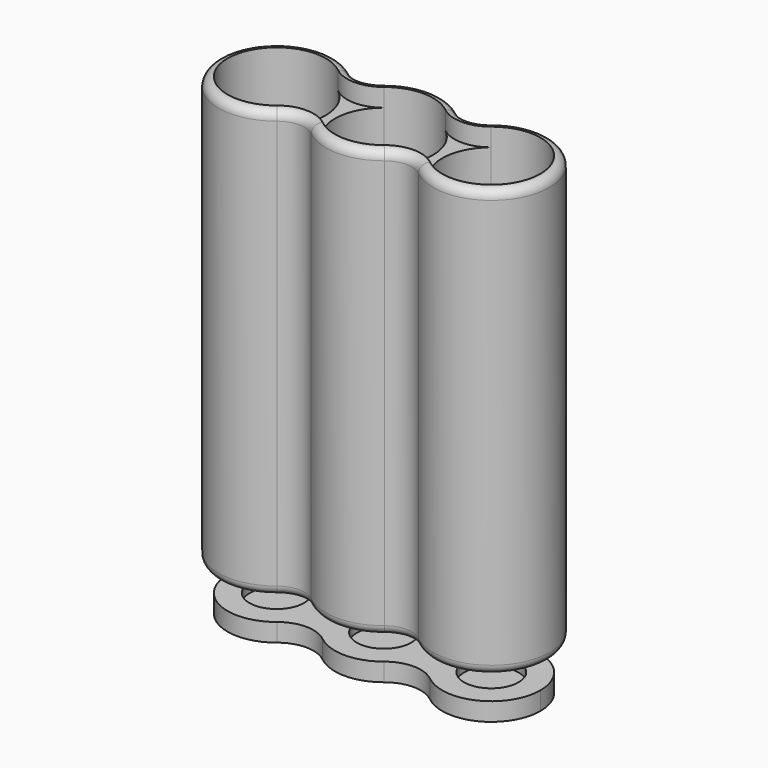
from build123d import *

# Parameters (mm, degrees)
F1_DEPTH = 47
F2_DEPTH = 45
F3_DEPTH = 1
F4_R     = 0.99999
F5_START = -3
F5_DEPTH = 2
F6_R     = 3
F7_DEPTH = 1


# Not quite as in the source:
# - a fillet or chamfer is up to 0.001 mm smaller than in the source, because OpenCascade refuses the exact size


with BuildPart() as f1:
    # F0 (on Top) → F1 (new body)
    with BuildSketch(Plane.XY):
        with BuildLine():
            ThreePointArc((4.0170212766, -4.9823227578), (5.9, -4.3177865506), (7.7829787234, -4.9823227578))
            ThreePointArc((7.7829787234, -4.9823227578), (11.8, -6.4), (15.8170212766, -4.9823227578))
            ThreePointArc((15.8170212766, -4.9823227578), (17.7, -4.3177865506), (19.5829787234, -4.9823227578))
            ThreePointArc((19.5829787234, -4.9823227578), (30, 0), (19.5829787234, 4.9823227578))
            ThreePointArc((19.5829787234, 4.9823227578), (17.7, 4.3177865506), (15.8170212766, 4.9823227578))
            ThreePointArc((15.8170212766, 4.9823227578), (11.8, 6.4), (7.7829787234, 4.9823227578))
            ThreePointArc((7.7829787234, 4.9823227578), (5.9, 4.3177865506), (4.0170212766, 4.9823227578))
            ThreePointArc((4.0170212766, 4.9823227578), (-6.4, 0), (4.0170212766, -4.9823227578))
        make_face()
        with BuildLine():
            ThreePointArc((3.3893617021, -4.2038348269), (-5.4, 0), (3.3893617021, 4.2038348269))
            ThreePointArc((3.3893617021, 4.2038348269), (5.9, 3.3177865506), (8.4106382979, 4.2038348269))
            ThreePointArc((8.4106382979, 4.2038348269), (11.8, 5.4), (15.1893617021, 4.2038348269))
            ThreePointArc((15.1893617021, 4.2038348269), (17.7, 3.3177865506), (20.2106382979, 4.2038348269))
            ThreePointArc((20.2106382979, 4.2038348269), (25.9299621036, 4.8714758129), (29, 0))
            ThreePointArc((29, 0), (25.9299621036, -4.8714758129), (20.2106382979, -4.2038348269))
            ThreePointArc((20.2106382979, -4.2038348269), (17.7, -3.3177865506), (15.1893617021, -4.2038348269))
            ThreePointArc((15.1893617021, -4.2038348269), (11.8, -5.4), (8.4106382979, -4.2038348269))
            ThreePointArc((8.4106382979, -4.2038348269), (5.9, -3.3177865506), (3.3893617021, -4.2038348269))
        make_face(mode=Mode.SUBTRACT)
    extrude(amount=F1_DEPTH)

    # F0 (on Top) → F2 (join)
    with BuildSketch(Plane.XY):
        with BuildLine():
            ThreePointArc((3.3893617021, 4.2038348269), (4.8714758129, 2.3299621036), (5.4, 0))
            ThreePointArc((5.4, 0), (4.8714758129, -2.3299621036), (3.3893617021, -4.2038348269))
            ThreePointArc((3.3893617021, -4.2038348269), (5.9, -3.3177865506), (8.4106382979, -4.2038348269))
            ThreePointArc((8.4106382979, -4.2038348269), (6.4, 0), (8.4106382979, 4.2038348269))
            ThreePointArc((8.4106382979, 4.2038348269), (5.9, 3.3177865506), (3.3893617021, 4.2038348269))
        make_face()
        with BuildLine():
            ThreePointArc((20.2106382979, 4.2038348269), (17.7, 3.3177865506), (15.1893617021, 4.2038348269))
            ThreePointArc((15.1893617021, 4.2038348269), (16.6714758129, 2.3299621036), (17.2, 0))
            ThreePointArc((17.2, 0), (16.6714758129, -2.3299621036), (15.1893617021, -4.2038348269))
            ThreePointArc((15.1893617021, -4.2038348269), (17.7, -3.3177865506), (20.2106382979, -4.2038348269))
            ThreePointArc((20.2106382979, -4.2038348269), (18.2, 0), (20.2106382979, 4.2038348269))
        make_face()
    extrude(amount=F2_DEPTH)

    # F0 (on Top) → F3 (join)
    with BuildSketch(Plane.XY):
        with BuildLine():
            ThreePointArc((3.3893617021, -4.2038348269), (4.8714758129, -2.3299621036), (5.4, 0))
            ThreePointArc((5.4, 0), (4.8714758129, 2.3299621036), (3.3893617021, 4.2038348269))
            ThreePointArc((3.3893617021, 4.2038348269), (-5.4, 0), (3.3893617021, -4.2038348269))
        make_face()
        with BuildLine():
            ThreePointArc((15.1893617021, 4.2038348269), (11.8, 5.4), (8.4106382979, 4.2038348269))
            ThreePointArc((8.4106382979, 4.2038348269), (6.4, 0), (8.4106382979, -4.2038348269))
            ThreePointArc((8.4106382979, -4.2038348269), (11.8, -5.4), (15.1893617021, -4.2038348269))
            ThreePointArc((15.1893617021, -4.2038348269), (16.6714758129, -2.3299621036), (17.2, 0))
            ThreePointArc((17.2, 0), (16.6714758129, 2.3299621036), (15.1893617021, 4.2038348269))
        make_face()
        with BuildLine():
            ThreePointArc((29, 0), (25.9299621036, 4.8714758129), (20.2106382979, 4.2038348269))
            ThreePointArc((20.2106382979, 4.2038348269), (18.2, 0), (20.2106382979, -4.2038348269))
            ThreePointArc((20.2106382979, -4.2038348269), (25.9299621036, -4.8714758129), (29, 0))
        make_face()
    extrude(amount=F3_DEPTH)

    # F4 (radius 1 in the source; OpenCascade refuses exactly that, so slightly less here)
    f4_edges = [f1.edges().sort_by_distance(p)[0] for p in [
        (11.8, 6.4, 47),
        (5.9, 4.317787, 47),
        (-6.4, 0, 47),
        (5.9, -4.317787, 47),
        (11.8, -6.4, 47),
        (17.7, -4.317787, 47),
        (30, 0, 47),
        (17.7, 4.317787, 47),
        (5.9, -4.317787, 0),
        (11.8, -6.4, 0),
        (17.7, -4.317787, 0),
        (30, 0, 0),
        (17.7, 4.317787, 0),
        (11.8, 6.4, 0),
        (5.9, 4.317787, 0),
        (-6.4, 0, 0),
    ]]
    fillet(f4_edges, radius=F4_R)


with BuildPart() as f5:
    # F0 (on Top) → F5 (new body)
    with BuildSketch(Plane.XY.offset(F5_START)):
        with BuildLine():
            ThreePointArc((3.3893617021, -4.2038348269), (4.8714758129, -2.3299621036), (5.4, 0))
            ThreePointArc((5.4, 0), (4.8714758129, 2.3299621036), (3.3893617021, 4.2038348269))
            ThreePointArc((3.3893617021, 4.2038348269), (-5.4, 0), (3.3893617021, -4.2038348269))
        make_face()
        with BuildLine():
            ThreePointArc((3.3893617021, 4.2038348269), (4.8714758129, 2.3299621036), (5.4, 0))
            ThreePointArc((5.4, 0), (4.8714758129, -2.3299621036), (3.3893617021, -4.2038348269))
            ThreePointArc((3.3893617021, -4.2038348269), (5.9, -3.3177865506), (8.4106382979, -4.2038348269))
            ThreePointArc((8.4106382979, -4.2038348269), (6.4, 0), (8.4106382979, 4.2038348269))
            ThreePointArc((8.4106382979, 4.2038348269), (5.9, 3.3177865506), (3.3893617021, 4.2038348269))
        make_face()
        with BuildLine():
            ThreePointArc((15.1893617021, 4.2038348269), (11.8, 5.4), (8.4106382979, 4.2038348269))
            ThreePointArc((8.4106382979, 4.2038348269), (6.4, 0), (8.4106382979, -4.2038348269))
            ThreePointArc((8.4106382979, -4.2038348269), (11.8, -5.4), (15.1893617021, -4.2038348269))
            ThreePointArc((15.1893617021, -4.2038348269), (16.6714758129, -2.3299621036), (17.2, 0))
            ThreePointArc((17.2, 0), (16.6714758129, 2.3299621036), (15.1893617021, 4.2038348269))
        make_face()
        with BuildLine():
            ThreePointArc((20.2106382979, 4.2038348269), (17.7, 3.3177865506), (15.1893617021, 4.2038348269))
            ThreePointArc((15.1893617021, 4.2038348269), (16.6714758129, 2.3299621036), (17.2, 0))
            ThreePointArc((17.2, 0), (16.6714758129, -2.3299621036), (15.1893617021, -4.2038348269))
            ThreePointArc((15.1893617021, -4.2038348269), (17.7, -3.3177865506), (20.2106382979, -4.2038348269))
            ThreePointArc((20.2106382979, -4.2038348269), (18.2, 0), (20.2106382979, 4.2038348269))
        make_face()
        with BuildLine():
            ThreePointArc((29, 0), (25.9299621036, 4.8714758129), (20.2106382979, 4.2038348269))
            ThreePointArc((20.2106382979, 4.2038348269), (18.2, 0), (20.2106382979, -4.2038348269))
            ThreePointArc((20.2106382979, -4.2038348269), (25.9299621036, -4.8714758129), (29, 0))
        make_face()
    extrude(amount=-F5_DEPTH)

    # F6 (on face) → F7 (cut)
    with BuildSketch(Plane.XY.offset(-3)):
        Circle(F6_R)
        with Locations((11.8, 0)):
            Circle(F6_R)
        with Locations((23.6, 0)):
            Circle(F6_R)
    extrude(amount=-F7_DEPTH, mode=Mode.SUBTRACT)


solid = Compound([f1.part, f5.part])
